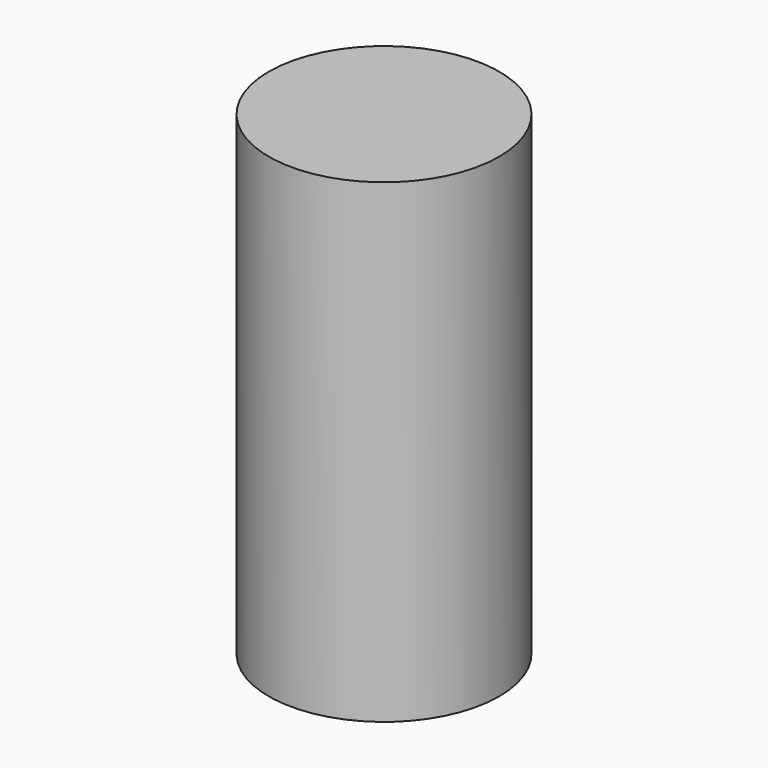
from build123d import *

# Parameters (mm, degrees)
F0_R     = 25.496477248
F1_DEPTH = 105.156


# Not quite as in the source:
# - the program builds the solid bodies; features that only make, move or delete a surface that nothing else refers to are left out


with BuildPart() as f1:
    # F0 (on Top) → F1 (new body)
    with BuildSketch(Plane.XY):
        Circle(F0_R)
    extrude(amount=F1_DEPTH)


solid = f1.part
